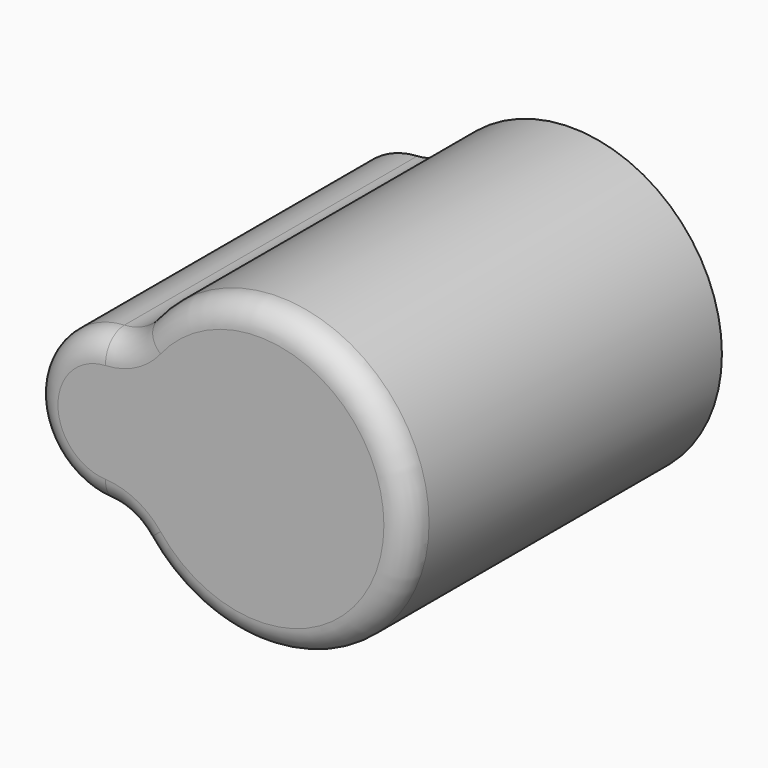
from build123d import *

# Parameters (mm, degrees)
F1_DEPTH = 78
F2_R     = 5


# Not quite as in the source:
# - a feature of the source that left no trace in its solid (it failed there, or was rolled back) is left out


with BuildPart() as f1:
    # F0 (on Front) → F1 (new body)
    with BuildSketch(Plane.XZ):
        with BuildLine():
            ThreePointArc((-30.75, -14.9812382666), (-26.6913543678, -16.0682388848), (-23.4375, -18.7265478332))
            ThreePointArc((-23.4375, -18.7265478332), (30, 0), (-23.4375, 18.7265478332))
            ThreePointArc((-23.4375, 18.7265478332), (-26.6913543678, 16.0682388848), (-30.75, 14.9812382666))
            ThreePointArc((-30.75, 14.9812382666), (-45, 0), (-30.75, -14.9812382666))
        make_face()
    extrude(amount=-F1_DEPTH)

    # F2
    f2_edges = [f1.edges().sort_by_distance(p)[0] for p in [
        (30, 0, 0),
        (-26.691354, 0, 16.068239),
        (-45, 0, 0),
        (-26.691354, 0, -16.068239),
    ]]
    fillet(f2_edges, radius=F2_R)


solid = f1.part
